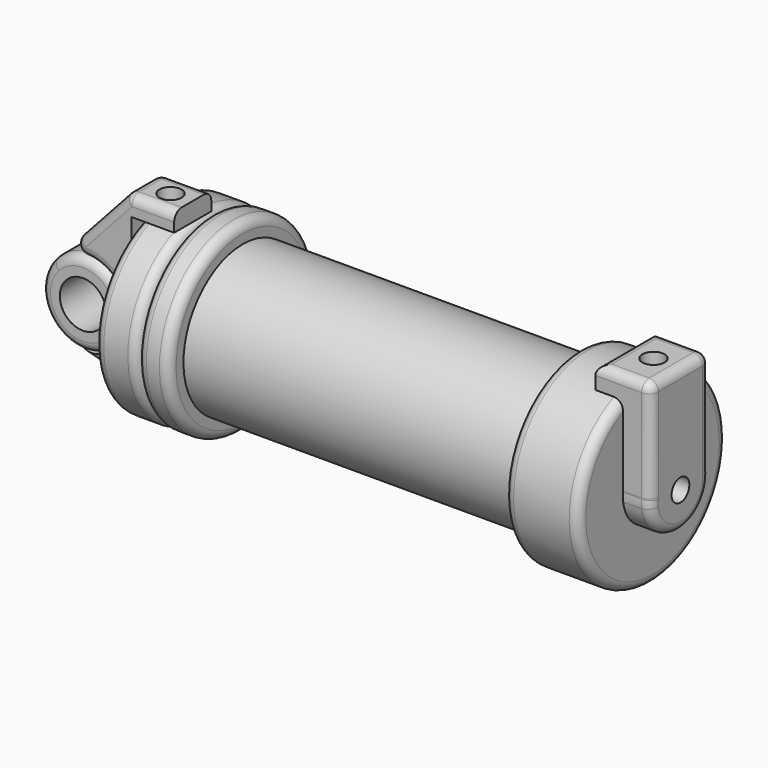
from build123d import *

# Parameters (mm, degrees)
F2_DEPTH  = 6.35
F0_W      = 5.842
F0_H      = 12.7
F4_DEPTH  = 6.35
F0_R      = 3.175
F5_DEPTH  = 6.35
F6_R      = 1.524
F7_DEPTH  = 3.81
F9_R      = 1.524
F10_DEPTH = 17.78
F8_R      = 1.524
F11_DEPTH = 10.414
F12_R     = 1.27
F12_2_R   = 1.27
F13_R     = 1.27
F14_R     = 1.27
F14_2_R   = 1.27
F14_3_R   = 1.27
F14_4_R   = 1.27
F14_5_R   = 1.27


with BuildPart() as f1:
    # F0 (on Front) → F1 (revolve)
    with BuildSketch(Plane.XZ):
        Polygon((5.842, 12.7), (5.842, 0), (66.294, 0), (66.294, 12.7), (56.134, 12.7), (56.134, 10.16), (10.16, 10.16), (10.16, 12.7), align=None)
    revolve(axis=Axis((33.147, 0, 0), (-1, 0, 0)))

    # F12
    f12_edges = [f1.edges().sort_by_distance(p)[0] for p in [
        (5.842, 0, -12.7),
    ]]
    fillet(f12_edges, radius=F12_R)

    # F13
    f13_edges = [f1.edges().sort_by_distance(p)[0] for p in [
        (66.294, 0, -12.7),
        (56.134, 0, -12.7),
    ]]
    fillet(f13_edges, radius=F13_R)

    # F14
    f14_edges = [f1.edges().sort_by_distance(p)[0] for p in [
        (10.16, 0, -12.7),
        (7.112, 0, -12.7),
    ]]
    fillet(f14_edges, radius=F14_R)


with BuildPart() as f2:
    # F0 (on Front) → F2 (new body)
    with BuildSketch(Plane.XZ):
        with BuildLine():
            Line((-0.9398, 0), (0, 0))
            Line((0, 0), (0, 12.7))
            Line((0, 12.7), (5.842, 12.7))
            Line((5.842, 12.7), (5.842, 15.24))
            Line((5.842, 15.24), (-0.508, 15.24))
            Line((-0.508, 15.24), (-10.8806298187, 3.8475430269))
            ThreePointArc((-10.8806298187, 3.8475430269), (-4.5919612295, 5.3297205562), (-0.9398, 0))
        make_face()
    extrude(amount=F2_DEPTH)

    # F9 (on face) → F10 (cut)
    with BuildSketch(Plane.XY.offset(15.24)):
        with Locations((2.9105336871, -3.3153819386)):
            Circle(F9_R)
    extrude(amount=-F10_DEPTH, mode=Mode.SUBTRACT)

    # F14#2
    f14_2_edges = [f2.edges().sort_by_distance(p)[0] for p in [
        (2.667, -6.35, 15.24),
        (-5.694315, 0, 9.543772),
        (-5.694315, -6.35, 9.543772),
        (-10.88063, -3.175, 3.847543),
        (-0.508, -3.175, 15.24),
        (2.667, 0, 15.24),
        (-4.591961, -6.35, 5.329721),
    ]]
    fillet(f14_2_edges, radius=F14_2_R)


with BuildPart() as f3:
    # F0 (on Front) → F3 (revolve)
    with BuildSketch(Plane.XZ):
        with Locations((2.921, 6.35)):
            Rectangle(F0_W, F0_H)
    revolve(axis=Axis((33.147, 0, 0), (-1, 0, 0)))

    # F14#3
    f14_3_edges = [f3.edges().sort_by_distance(p)[0] for p in [
        (5.842, 0, -12.7),
        (0, 0, -12.7),
    ]]
    fillet(f14_3_edges, radius=F14_3_R)


with BuildPart() as f4:
    # F0 (on Front) → F4 (new body)
    with BuildSketch(Plane.XZ):
        with BuildLine():
            Line((5.842, 0), (0, 0))
            Line((0, 0), (-0.9398, 0))
            ThreePointArc((-0.9398, 0), (-3.1957909266, -4.5493385486), (-8.1826630726, -5.5069827884))
            Line((-8.1826630726, -5.5069827884), (5.842, -9.398))
            Line((5.842, -9.398), (5.842, 0))
        make_face()
    extrude(amount=F4_DEPTH)

    # F14#4
    f14_4_edges = [f4.edges().sort_by_distance(p)[0] for p in [
        (-1.170332, -6.35, -7.452491),
    ]]
    fillet(f14_4_edges, radius=F14_4_R)


with BuildPart() as f5:
    # F0 (on Front) → F5 (new body)
    with BuildSketch(Plane.XZ):
        with BuildLine():
            ThreePointArc((-8.1826630726, -5.5069827884), (-3.1957909266, -4.5493385486), (-0.9398, 0))
            ThreePointArc((-0.9398, 0), (-4.5919612295, 5.3297205562), (-10.8806298187, 3.8475430269))
            ThreePointArc((-10.8806298187, 3.8475430269), (-12.1459778134, -1.5837270034), (-8.1826630726, -5.5069827884))
        make_face()
        with Locations((-6.6548, 0)):
            Circle(F0_R, mode=Mode.SUBTRACT)
    extrude(amount=F5_DEPTH)

    # F14#5
    f14_5_edges = [f5.edges().sort_by_distance(p)[0] for p in [
        (-2.42897, -6.35, -3.847543),
    ]]
    fillet(f14_5_edges, radius=F14_5_R)


with BuildPart() as f7:
    # F6 (on face) → F7 (new body, symmetric)
    with BuildSketch(Plane.YZ.offset(66.294)):
        with BuildLine():
            Line((-5.0444914745, 0.5995879951), (-5.0444914745, -0.5995879951))
            ThreePointArc((-5.0444914745, -0.5995879951), (0, -5.08), (5.0444914745, -0.5995879951))
            Line((5.0444914745, -0.5995879951), (5.0444914745, 0.5995879951))
            ThreePointArc((5.0444914745, 0.5995879951), (0, 5.08), (-5.0444914745, 0.5995879951))
        make_face()
        Circle(F6_R, mode=Mode.SUBTRACT)
        with BuildLine():
            ThreePointArc((-5.0444914745, 0.5995879951), (-5.08, 0), (-5.0444914745, -0.5995879951))
            Line((-5.0444914745, -0.5995879951), (-5.0444914745, 0.5995879951))
        make_face()
        with BuildLine():
            Line((5.0444914745, 0.5995879951), (5.0444914745, -0.5995879951))
            ThreePointArc((5.0444914745, -0.5995879951), (5.0711150988, -0.3003192548), (5.08, 0))
            ThreePointArc((5.08, 0), (5.0711150988, 0.3003192548), (5.0444914745, 0.5995879951))
        make_face()
        with BuildLine():
            Line((-5.0444914745, 14.6404120049), (-5.0444914745, 0.5995879951))
            ThreePointArc((-5.0444914745, 0.5995879951), (0, 5.08), (5.0444914745, 0.5995879951))
            Line((5.0444914745, 0.5995879951), (5.0444914745, 14.6404120049))
            Line((5.0444914745, 14.6404120049), (-5.0444914745, 14.6404120049))
        make_face()
    extrude(amount=F7_DEPTH, both=True)

    # F8 (on face) → F11 (cut)
    with BuildSketch(Plane.XY.offset(14.6404120049)):
        with Locations((66.3770288229, 0.0502656185)):
            Circle(F8_R)
    extrude(amount=-F11_DEPTH, mode=Mode.SUBTRACT)

    # F12#2
    f12_2_edges = [f7.edges().sort_by_distance(p)[0] for p in [
        (70.104, -5.044491, 7.62),
        (70.104, 5.044491, 7.62),
        (70.104, 0, -5.08),
        (70.104, 0, 14.640412),
        (66.294, 5.044491, 14.640412),
        (66.294, -5.044491, 14.640412),
        (62.484, 0, 14.640412),
        (66.294, -5.044491, 0.599588),
    ]]
    fillet(f12_2_edges, radius=F12_2_R)


solid = Compound([f1.part, f2.part, f3.part, f4.part, f5.part, f7.part])
